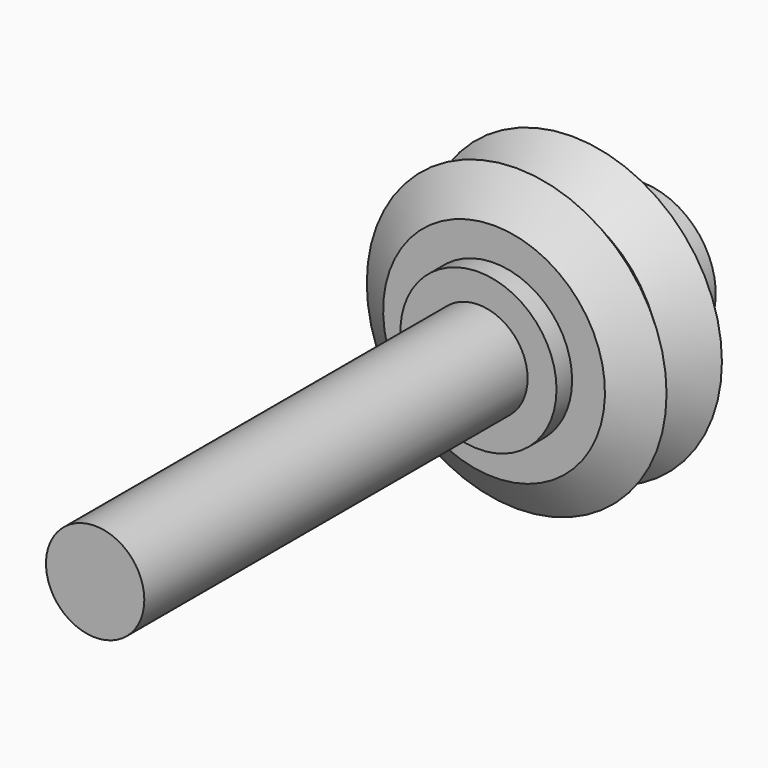
from build123d import *

# Parameters (mm, degrees)
F2_R     = 6.35
F2_R_2   = 4
F3_DEPTH = 1.5875
F4_R     = 6.0423658591
F5_DEPTH = 4.7625
F6_R     = 4
F7_DEPTH = 50.8


with BuildPart() as f1:
    # F0 (on Right) → F1 (revolve)
    with BuildSketch(Plane.YZ):
        Polygon((-5.115, 9.0238079429), (-5.115, 4), (5.115, 4), (5.115, 9.0238079429), (2.815, 12.195), (0, 9.38), (-2.815, 12.195), align=None)
    revolve(axis=Axis((0, -0.9241095702, 0), (0, 1, 0)))


with BuildPart() as f3:
    # F2 (on face) → F3 (new body)
    with BuildSketch(Plane.XZ.offset(5.115)):
        Circle(F2_R)
        Circle(F2_R_2, mode=Mode.SUBTRACT)
    extrude(amount=F3_DEPTH)


with BuildPart() as f5:
    # F4 (on face) → F5 (new body)
    with BuildSketch(Plane(origin=(0, 5.115, 0), x_dir=(-1, 0, 0), z_dir=(0, 1, 0))):
        Circle(F4_R)
    extrude(amount=F5_DEPTH)

    # F6 (on face) → F7 (join)
    with BuildSketch(Plane.XZ.offset(-5.115)):
        Circle(F6_R)
    extrude(amount=F7_DEPTH)


solid = Compound([f1.part, f3.part, f5.part])
